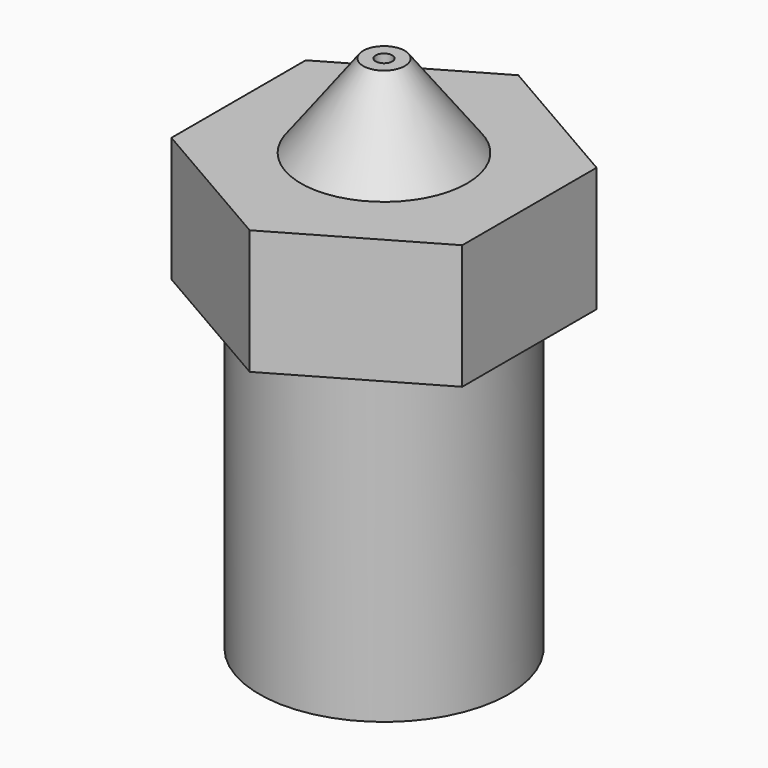
from build123d import *

# Parameters (mm, degrees)
F1_R      = 3
F2_DEPTH  = 7.5
F3_R      = 3
F4_DEPTH  = 3
F5_R      = 2
F6_DEPTH  = 2
F7_SIZE2  = 1.99999
F7_SIZE   = 1.49999
F8_D      = 0.4
F10_D     = 2.5
F10_DEPTH = 5
F10_TIP   = 0.7510757738


# Not quite as in the source:
# - a fillet or chamfer is up to 0.001 mm smaller than in the source, because OpenCascade refuses the exact size


with BuildPart() as f2:
    # F1 (on face) → F2 (new body)
    with BuildSketch(Plane.XY):
        Circle(F1_R)
    extrude(amount=F2_DEPTH)

    # F3 (on face) → F4 (join)
    with BuildSketch(Plane.XY.offset(7.5)):
        Polygon((3.5, -2.0207259422), (3.5, 2.0207259422), (0, 4.0414518843), (-3.5, 2.0207259422), (-3.5, -2.0207259422), (0, -4.0414518843), align=None)
        Circle(F3_R, mode=Mode.SUBTRACT)
        Circle(F3_R)
    extrude(amount=F4_DEPTH)

    # F5 (on face) → F6 (join)
    with BuildSketch(Plane.XY.offset(10.5)):
        Circle(F5_R)
    extrude(amount=F6_DEPTH)

    # F7 (size 1.5 and 2 in the source; OpenCascade refuses exactly that, so slightly less here)
    f7_edges = [f2.edges().sort_by_distance(p)[0] for p in [
        (-2, 0, 12.5),
    ]]
    f7_side = f2.faces().sort_by_distance((0, 0, 12.5))[0]
    chamfer(f7_edges, length=F7_SIZE, length2=F7_SIZE2, reference=f7_side)

    # F8 (through all)
    with Locations(Plane(origin=(0, 0, 0), x_dir=(1, 0, 0), z_dir=(0, 0, -1))):
        with Locations((0, 0)):
            Hole(F8_D / 2)

    # F10
    with Locations(Plane(origin=(0, 0, 0), x_dir=(1, 0, 0), z_dir=(0, 0, -1))):
        with Locations((0, 0)):
            Hole(F10_D / 2, depth=F10_DEPTH)
            with Locations((0, 0, -(F10_DEPTH + F10_TIP / 2))):  # 118° drill point
                Cone(0, F10_D / 2, F10_TIP, mode=Mode.SUBTRACT)


solid = f2.part
